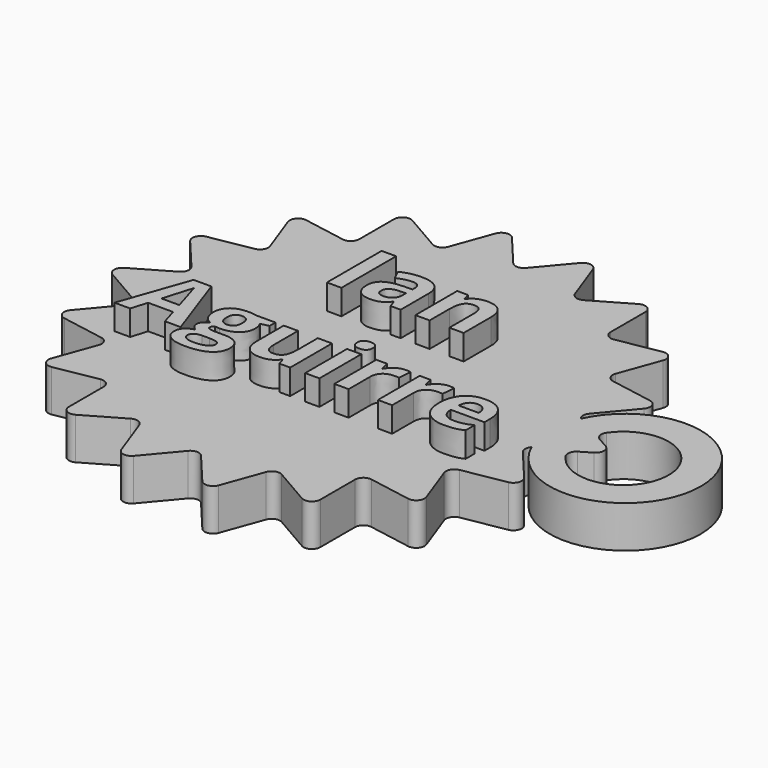
from build123d import *

# Parameters (mm, degrees)
F1_DEPTH      = 5
F2_R          = 1
F3_R          = 1
F4_R          = 9.02426598
F5_DEPTH      = 5
F7_DEPTH      = 5
F8_R          = 1
F10_DEPTH     = 4.5
F11_R         = 7.0893465871
F11_R_2       = 5.3736476411
F12_DEPTH     = 4.5
F13_TEXT_SIZE = 11.4339189247
F14_DEPTH     = 3


# Not quite as in the source:
# - a feature names something its author has since deleted; it is built from what else it names
# - Text() gives the source's letters only with a copy of the font that has no kerning and outlines rounded to 1/6400 em; it was checked with that copy


with BuildPart() as f1:
    # F0 (on Top) → F1 (new body)
    with BuildSketch(Plane.XY):
        Polygon((-69.4327632519, 10.2606042998), (-64.2233179219, 4.0522291123), (-71.2419846284, 0), (-64.2233179219, -4.0522291123), (-69.4327632519, -10.2606042998), (-61.4514299584, -11.6679287015), (-64.2233179219, -19.2836282906), (-56.2419846284, -17.8763038889), (-56.2419846284, -25.9807621135), (-49.2233179219, -21.9285330012), (-46.4514299584, -29.5442325904), (-41.2419846284, -23.3358574029), (-36.0325392983, -29.5442325904), (-33.2606513348, -21.9285330012), (-26.2419846284, -25.9807621135), (-26.2419846284, -17.8763038889), (-18.2606513348, -19.2836282906), (-21.0325392984, -11.6679287015), (-13.0512060048, -10.2606042998), (-18.2606513348, -4.0522291123), (-11.2419846284, 0), (-18.2606513348, 4.0522291123), (-13.0512060048, 10.2606042998), (-21.0325392984, 11.6679287015), (-18.2606513348, 19.2836282906), (-26.2419846284, 17.8763038889), (-26.2419846284, 25.9807621135), (-33.2606513348, 21.9285330012), (-36.0325392984, 29.5442325904), (-41.2419846284, 23.3358574029), (-46.4514299584, 29.5442325904), (-49.2233179219, 21.9285330012), (-56.2419846284, 25.9807621135), (-56.2419846284, 17.8763038889), (-64.2233179219, 19.2836282906), (-61.4514299584, 11.6679287015), align=None)
    extrude(amount=F1_DEPTH)

    # F2
    f2_edges = [f1.edges().sort_by_distance(p)[0] for p in [
        (-49.223318, -21.928533, 2.5),
        (-56.241985, -17.876304, 2.5),
        (-61.45143, -11.667929, 2.5),
        (-64.223318, -4.052229, 2.5),
        (-64.223318, 4.052229, 2.5),
        (-61.45143, 11.667929, 2.5),
        (-56.241985, 17.876304, 2.5),
        (-49.223318, 21.928533, 2.5),
        (-41.241985, 23.335857, 2.5),
        (-33.260651, 21.928533, 2.5),
        (-41.241985, -23.335857, 2.5),
        (-33.260651, -21.928533, 2.5),
        (-26.241985, -17.876304, 2.5),
        (-21.032539, -11.667929, 2.5),
        (-26.241985, 17.876304, 2.5),
        (-21.032539, 11.667929, 2.5),
        (-18.260651, 4.052229, 2.5),
        (-18.260651, -4.052229, 2.5),
    ]]
    fillet(f2_edges, radius=F2_R)

    # F3
    f3_edges = [f1.edges().sort_by_distance(p)[0] for p in [
        (-36.032539, 29.544233, 2.5),
        (-26.241985, 25.980762, 2.5),
        (-18.260651, 19.283628, 2.5),
        (-13.051206, 10.260604, 2.5),
        (-11.241985, 0, 2.5),
        (-13.051206, -10.260604, 2.5),
        (-56.241985, 25.980762, 2.5),
        (-46.45143, 29.544233, 2.5),
        (-64.223318, 19.283628, 2.5),
        (-69.432763, 10.260604, 2.5),
        (-71.241985, 0, 2.5),
        (-69.432763, -10.260604, 2.5),
        (-64.223318, -19.283628, 2.5),
        (-56.241985, -25.980762, 2.5),
        (-46.45143, -29.544233, 2.5),
        (-36.032539, -29.544233, 2.5),
        (-26.241985, -25.980762, 2.5),
        (-18.260651, -19.283628, 2.5),
    ]]
    fillet(f3_edges, radius=F3_R)

    # F4 (on Top) → F5 (join, through all)
    with BuildSketch(Plane.XY):
        with Locations((-9.2419846284, 0)):
            Circle(F4_R)
    extrude(amount=F5_DEPTH)

    # F6 (on face) → F7 (cut, through all)
    with BuildSketch(Plane.XY.offset(5)):
        with BuildLine():
            ThreePointArc((-14.3705448136, -2.1852792706), (-3.981082649, -0.0942598595), (-14.3705448136, 1.9967595517))
            Line((-14.3705448136, 1.9967595517), (-10.7515631244, 0))
            Line((-10.7515631244, 0), (-14.3705448136, -2.1852792706))
        make_face()
    extrude(amount=-F7_DEPTH, mode=Mode.SUBTRACT)

    # F8
    f8_edges = [f1.edges().sort_by_distance(p)[0] for p in [
        (-10.751563, 0, 2.5),
        (-14.370545, -2.185279, 2.5),
        (-14.370545, 1.99676, 2.5),
    ]]
    fillet(f8_edges, radius=F8_R)

    # F9 (on face) → F10 (cut)
    with BuildSketch(Plane.XY):
        with BuildLine():
            ThreePointArc((-35.3777156799, -4.6599307489), (-35.5753046169, -4.908160303), (-35.7829730175, -5.1480209603))
            Line((-35.7829730175, -5.1480209603), (-21.9766725259, -17.609254409))
            Line((-21.9766725259, -17.609254409), (-20.5904544794, -15.9396992978))
            Line((-20.5904544794, -15.9396992978), (-35.3777156799, -4.6599307489))
        make_face()
        with BuildLine():
            Line((-35.0430152336, -4.1849240607), (-22.1269458204, -12.5734481191))
            Line((-22.1269458204, -12.5734481191), (-20.8090839907, -10.2629405882))
            Line((-20.8090839907, -10.2629405882), (-34.6043804511, -3.4158988524))
            ThreePointArc((-34.6043804511, -3.4158988524), (-34.8126121734, -3.8067344742), (-35.0430152336, -4.1849240607))
        make_face()
        with BuildLine():
            ThreePointArc((-34.1823081919, -2.3833949122), (-34.2698744439, -2.6366901562), (-34.3662212872, -2.8867773708))
            Line((-34.3662212872, -2.8867773708), (-17.1305497448, -9.8744736155))
            Line((-17.1305497448, -9.8744736155), (-16.3989523541, -7.8314905025))
            Line((-16.3989523541, -7.8314905025), (-19.4509472573, -6.8787666419))
            Line((-19.4509472573, -6.8787666419), (-34.1823081919, -2.3833949122))
        make_face()
        with BuildLine():
            Line((-34.0002869576, -1.7286818538), (-18.9941076397, -5.1937600989))
            Line((-18.9941076397, -5.1937600989), (-18.54596272, -2.5718579299))
            Line((-18.54596272, -2.5718579299), (-33.8511272013, -0.8560126092))
            ThreePointArc((-33.8511272013, -0.8560126092), (-33.9131273587, -1.2944974025), (-34.0002869576, -1.7286818538))
        make_face()
        with BuildLine():
            ThreePointArc((-33.8115942061, 0.3570473634), (-33.8033972316, 0.0398847724), (-33.8083009973, -0.2773458261))
            Line((-33.8083009973, -0.2773458261), (-15.2221347635, -0.9486855723))
            Line((-15.2221347635, -0.9486855723), (-15.2333994712, 1.2213116278))
            Line((-15.2333994712, 1.2213116278), (-33.8115942061, 0.3570473634))
        make_face()
        with BuildLine():
            Line((-33.8605272028, 0.9360648973), (-18.5742046736, 2.812372041))
            Line((-18.5742046736, 2.812372041), (-19.0498295551, 5.4294287513))
            Line((-19.0498295551, 5.4294287513), (-34.0188333405, 1.807121388))
            ThreePointArc((-34.0188333405, 1.807121388), (-33.9271237992, 1.3738751607), (-33.8605272028, 0.9360648973))
        make_face()
        with BuildLine():
            ThreePointArc((-34.3965754224, 2.9605459736), (-34.2803967911, 2.6653141576), (-34.1765055688, 2.3655377184))
            Line((-34.1765055688, 2.3655377184), (-16.481610594, 8.0915279521))
            Line((-16.481610594, 8.0915279521), (-17.2343787101, 10.1268055511))
            Line((-17.2343787101, 10.1268055511), (-34.3965754224, 2.9605459736))
        make_face()
        with BuildLine():
            Line((-34.6405930582, 3.4879084069), (-20.9178834168, 10.4792906065))
            Line((-20.9178834168, 10.4792906065), (-22.2599107194, 12.7758461952))
            Line((-22.2599107194, 12.7758461952), (-35.0872710335, 4.2522898756))
            ThreePointArc((-35.0872710335, 4.2522898756), (-34.8529133175, 3.8765381033), (-34.6405930582, 3.4879084069))
        make_face()
        with BuildLine():
            ThreePointArc((-35.8367269225, 5.2069590463), (-35.6265794919, 4.9692673195), (-35.4264240963, 4.7231025025))
            Line((-35.4264240963, 4.7231025025), (-20.7570658633, 16.1557837872))
            Line((-20.7570658633, 16.1557837872), (-22.1605424433, 17.8108572693))
            Line((-22.1605424433, 17.8108572693), (-35.8367269225, 5.2069590463))
        make_face()
        with BuildLine():
            Line((-36.2463970692, 5.6190586866), (-25.742461624, 16.882252067))
            Line((-25.742461624, 16.882252067), (-27.7890230487, 18.5813080366))
            Line((-27.7890230487, 18.5813080366), (-36.927570926, 6.184569447))
            ThreePointArc((-36.927570926, 6.184569447), (-36.5788320346, 5.911633339), (-36.2463970692, 5.6190586866))
        make_face()
        with BuildLine():
            ThreePointArc((-37.958345181, 6.8253360115), (-37.6795758328, 6.6738535042), (-37.4072979585, 6.5109914192))
            Line((-37.4072979585, 6.5109914192), (-27.5328175668, 22.2714136636))
            Line((-27.5328175668, 22.2714136636), (-29.4177226221, 23.3466567405))
            Line((-29.4177226221, 23.3466567405), (-37.958345181, 6.8253360115))
        make_face()
        with BuildLine():
            Line((-38.4842555729, 7.0724675602), (-32.4660239601, 21.2489647728))
            Line((-32.4660239601, 21.2489647728), (-34.9702739951, 22.1455898979))
            Line((-34.9702739951, 22.1455898979), (-39.3177656909, 7.3708986687))
            ThreePointArc((-39.3177656909, 7.3708986687), (-38.8967086813, 7.2336983476), (-38.4842555729, 7.0724675602))
        make_face()
        with BuildLine():
            ThreePointArc((-40.5055317243, 7.6204767225), (-40.191764156, 7.5734744606), (-39.8802045331, 7.5135586787))
            Line((-39.8802045331, 7.5135586787), (-35.9916100498, 25.7007823611))
            Line((-35.9916100498, 25.7007823611), (-38.1305962124, 26.0665048489))
            Line((-38.1305962124, 26.0665048489), (-40.5055317243, 7.6204767225))
        make_face()
        with BuildLine():
            Line((-41.0842498064, 7.6728324676), (-40.2776095782, 23.0527387256))
            Line((-40.2776095782, 23.0527387256), (-42.9374987105, 23.0387867834))
            Line((-42.9374987105, 23.0387867834), (-41.9695625642, 7.668188728))
            ThreePointArc((-41.9695625642, 7.668188728), (-41.5269731258, 7.6832725775), (-41.0842498064, 7.6728324676))
        make_face()
        with BuildLine():
            ThreePointArc((-43.1710582627, 7.4964754745), (-42.8601374738, 7.5596226245), (-42.5468747909, 7.6098798733))
            Line((-42.5468747909, 7.6098798733), (-45.1131881003, 26.0302574027))
            Line((-45.1131881003, 26.0302574027), (-47.2482620709, 25.6423477718))
            Line((-47.2482620709, 25.6423477718), (-43.1710582627, 7.4964754745))
        make_face()
        with BuildLine():
            Line((-43.7327820934, 7.3477405404), (-48.235025966, 22.0760121659))
            Line((-48.235025966, 22.0760121659), (-50.7297323105, 21.1531659665))
            Line((-50.7297323105, 21.1531659665), (-44.5631157065, 7.0405820563))
            ThreePointArc((-44.5631157065, 7.0405820563), (-44.1523766576, 7.2061307415), (-43.7327820934, 7.3477405404))
        make_face()
        with BuildLine():
            ThreePointArc((-45.6334229567, 6.468288648), (-45.362850583, 6.6339687317), (-45.085668943, 6.7883372453))
            Line((-45.085668943, 6.7883372453), (-53.7973547852, 23.2200992358))
            Line((-53.7973547852, 23.2200992358), (-55.6709951327, 22.1253451128))
            Line((-55.6709951327, 22.1253451128), (-45.6334229567, 6.468288648))
        make_face()
        with BuildLine():
            Line((-46.1104003519, 6.1364026629), (-55.3784912683, 18.4365927318))
            Line((-55.3784912683, 18.4365927318), (-57.4071164218, 16.7161611466))
            Line((-57.4071164218, 16.7161611466), (-46.7856043321, 5.5637772807))
            ThreePointArc((-46.7856043321, 5.5637772807), (-46.4562568639, 5.8598231869), (-46.1104003519, 6.1364026629))
        make_face()
        with BuildLine():
            ThreePointArc((-47.5956282836, 4.6599307489), (-47.3980393467, 4.908160303), (-47.190370946, 5.1480209603))
            Line((-47.190370946, 5.1480209603), (-60.9966714376, 17.609254409))
            Line((-60.9966714376, 17.609254409), (-62.3828894841, 15.9396992978))
            Line((-62.3828894841, 15.9396992978), (-47.5956282836, 4.6599307489))
        make_face()
        with BuildLine():
            Line((-47.93032873, 4.1849240607), (-60.8463981431, 12.5734481191))
            Line((-60.8463981431, 12.5734481191), (-62.1642599729, 10.2629405882))
            Line((-62.1642599729, 10.2629405882), (-48.3689635124, 3.4158988524))
            ThreePointArc((-48.3689635124, 3.4158988524), (-48.1607317901, 3.8067344742), (-47.93032873, 4.1849240607))
        make_face()
        with BuildLine():
            ThreePointArc((-48.821003322, 2.2895164282), (-48.7202299636, 2.590355305), (-48.6071226764, 2.8867773708))
            Line((-48.6071226764, 2.8867773708), (-65.8427942188, 9.8744736155))
            Line((-65.8427942188, 9.8744736155), (-66.5743916094, 7.8314905025))
            Line((-66.5743916094, 7.8314905025), (-48.821003322, 2.2895164282))
        make_face()
        with BuildLine():
            Line((-48.973057006, 1.7286818538), (-63.9792363238, 5.1937600989))
            Line((-63.9792363238, 5.1937600989), (-64.4273812436, 2.5718579299))
            Line((-64.4273812436, 2.5718579299), (-49.1222167623, 0.8560126092))
            ThreePointArc((-49.1222167623, 0.8560126092), (-49.0602166048, 1.2944974025), (-48.973057006, 1.7286818538))
        make_face()
        Polygon((-49.1617497575, -0.3570473634), (-49.1650429663, 0.2773458261), (-67.7512092001, 0.9486855723), (-67.7399444924, -1.2213116278), align=None)
        with BuildLine():
            ThreePointArc((-48.5767685411, -2.9605459736), (-48.6929471725, -2.6653141576), (-48.7968383947, -2.3655377184))
            Line((-48.7968383947, -2.3655377184), (-66.4917333696, -8.0915279521))
            Line((-66.4917333696, -8.0915279521), (-65.7389652535, -10.1268055511))
            Line((-65.7389652535, -10.1268055511), (-48.5767685411, -2.9605459736))
        make_face()
        with BuildLine():
            Line((-49.1128167608, -0.9360648973), (-64.39913929, -2.812372041))
            Line((-64.39913929, -2.812372041), (-63.9235144085, -5.4294287513))
            Line((-63.9235144085, -5.4294287513), (-48.954510623, -1.807121388))
            ThreePointArc((-48.954510623, -1.807121388), (-49.0462201644, -1.3738751607), (-49.1128167608, -0.9360648973))
        make_face()
        with BuildLine():
            Line((-48.3327509053, -3.4879084069), (-62.0554605467, -10.4792906065))
            Line((-62.0554605467, -10.4792906065), (-60.7134332442, -12.7758461952))
            Line((-60.7134332442, -12.7758461952), (-47.88607293, -4.2522898756))
            ThreePointArc((-47.88607293, -4.2522898756), (-48.1204306461, -3.8765381033), (-48.3327509053, -3.4879084069))
        make_face()
        with BuildLine():
            ThreePointArc((-47.1366170411, -5.2069590463), (-47.3467644716, -4.9692673195), (-47.5469198672, -4.7231025025))
            Line((-47.5469198672, -4.7231025025), (-62.2162781003, -16.1557837872))
            Line((-62.2162781003, -16.1557837872), (-60.8128015203, -17.8108572693))
            Line((-60.8128015203, -17.8108572693), (-47.1366170411, -5.2069590463))
        make_face()
        with BuildLine():
            Line((-46.7269468943, -5.6190586866), (-57.2308823396, -16.882252067))
            Line((-57.2308823396, -16.882252067), (-55.1843209149, -18.5813080366))
            Line((-55.1843209149, -18.5813080366), (-46.0457730376, -6.184569447))
            ThreePointArc((-46.0457730376, -6.184569447), (-46.394511929, -5.911633339), (-46.7269468943, -5.6190586866))
        make_face()
        with BuildLine():
            ThreePointArc((-45.0149987825, -6.8253360115), (-45.2937681308, -6.6738535042), (-45.566046005, -6.5109914192))
            Line((-45.566046005, -6.5109914192), (-55.4405263967, -22.2714136636))
            Line((-55.4405263967, -22.2714136636), (-53.5556213415, -23.3466567405))
            Line((-53.5556213415, -23.3466567405), (-45.0149987825, -6.8253360115))
        make_face()
        with BuildLine():
            Line((-44.4890883907, -7.0724675602), (-50.5073200035, -21.2489647728))
            Line((-50.5073200035, -21.2489647728), (-48.0030699685, -22.1455898979))
            Line((-48.0030699685, -22.1455898979), (-43.6555782727, -7.3708986687))
            ThreePointArc((-43.6555782727, -7.3708986687), (-44.0766352823, -7.2336983476), (-44.4890883907, -7.0724675602))
        make_face()
        with BuildLine():
            ThreePointArc((-42.4678122393, -7.6204767225), (-42.7815798076, -7.5734744606), (-43.0931394305, -7.5135586787))
            Line((-43.0931394305, -7.5135586787), (-46.9817339137, -25.7007823611))
            Line((-46.9817339137, -25.7007823611), (-44.8427477512, -26.0665048489))
            Line((-44.8427477512, -26.0665048489), (-42.4678122393, -7.6204767225))
        make_face()
        with BuildLine():
            Line((-41.8890941571, -7.6728324676), (-42.6957343854, -23.0527387256))
            Line((-42.6957343854, -23.0527387256), (-40.0358452531, -23.0387867834))
            Line((-40.0358452531, -23.0387867834), (-41.0037813994, -7.668188728))
            ThreePointArc((-41.0037813994, -7.668188728), (-41.4463708377, -7.6832725775), (-41.8890941571, -7.6728324676))
        make_face()
        with BuildLine():
            ThreePointArc((-39.8022857009, -7.4964754745), (-40.1132064898, -7.5596226245), (-40.4264691727, -7.6098798733))
            Line((-40.4264691727, -7.6098798733), (-37.8601558633, -26.0302574027))
            Line((-37.8601558633, -26.0302574027), (-35.7250818926, -25.6423477718))
            Line((-35.7250818926, -25.6423477718), (-39.8022857009, -7.4964754745))
        make_face()
        with BuildLine():
            Line((-39.2405618701, -7.3477405404), (-34.7383179975, -22.0760121659))
            Line((-34.7383179975, -22.0760121659), (-32.2436116531, -21.1531659665))
            Line((-32.2436116531, -21.1531659665), (-38.4102282571, -7.0405820563))
            ThreePointArc((-38.4102282571, -7.0405820563), (-38.8209673059, -7.2061307415), (-39.2405618701, -7.3477405404))
        make_face()
        with BuildLine():
            ThreePointArc((-37.3399210068, -6.468288648), (-37.6104933805, -6.6339687317), (-37.8876750206, -6.7883372453))
            Line((-37.8876750206, -6.7883372453), (-29.1759891784, -23.2200992358))
            Line((-29.1759891784, -23.2200992358), (-27.3023488309, -22.1253451128))
            Line((-27.3023488309, -22.1253451128), (-37.3399210068, -6.468288648))
        make_face()
        with BuildLine():
            Line((-36.8629436116, -6.1364026629), (-27.5948526953, -18.4365927318))
            Line((-27.5948526953, -18.4365927318), (-25.5662275418, -16.7161611466))
            Line((-25.5662275418, -16.7161611466), (-36.1877396314, -5.5637772807))
            ThreePointArc((-36.1877396314, -5.5637772807), (-36.5170870997, -5.8598231869), (-36.8629436116, -6.1364026629))
        make_face()
    extrude(amount=F10_DEPTH, mode=Mode.SUBTRACT)

    # F11 (on face) → F12 (cut, through all)
    with BuildSketch(Plane.XY):
        with Locations((-41.4866719818, 0)):
            Circle(F11_R)
        with Locations((-41.4866719818, 0)):
            Circle(F11_R_2, mode=Mode.SUBTRACT)
    extrude(amount=F12_DEPTH, mode=Mode.SUBTRACT)

    # F13 (on face) → F14 (join)
    with BuildSketch(Plane.XY.offset(5)):
        with Locations((-50.5703675708, 5.8652958457)):
            Text('Ian', F13_TEXT_SIZE, font='Open Sans', font_style=FontStyle.BOLD, text_align=(TextAlign.LEFT, TextAlign.BOTTOM))
        with Locations((-62.4544970531, -9.6848338919)):
            Text('Aguirre', F13_TEXT_SIZE, font='Open Sans', font_style=FontStyle.BOLD, text_align=(TextAlign.LEFT, TextAlign.BOTTOM))
    extrude(amount=F14_DEPTH)


solid = f1.part
